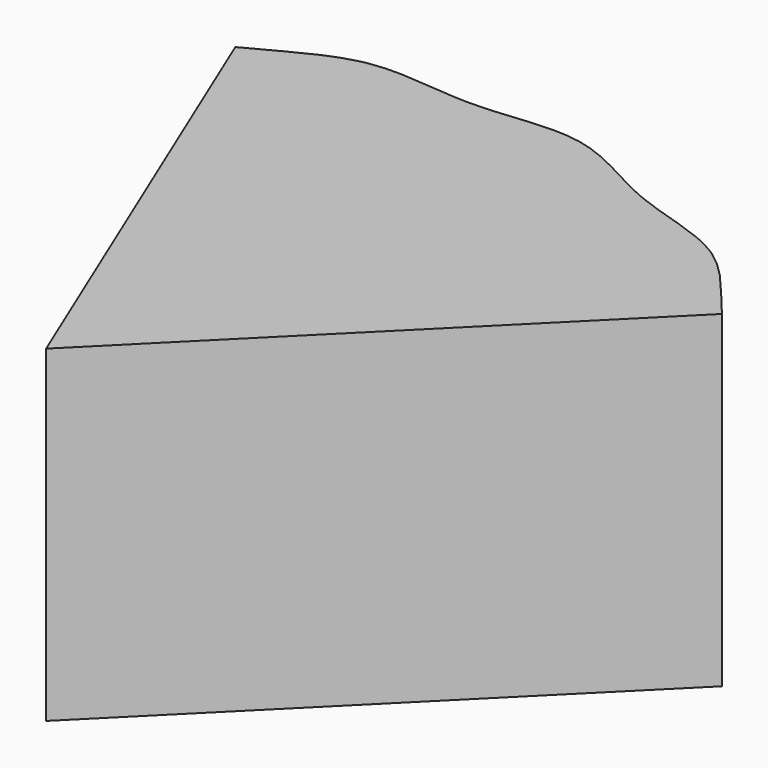
from build123d import *

# Parameters (mm, degrees)
F1_DEPTH = 25


# Not quite as in the source:
# - ends of sketch curves that miss each other by under 0.0002 mm in the source are joined


with BuildPart() as f1:
    # F0 (on Top) → F1 (new body)
    with BuildSketch(Plane.XY):
        with BuildLine():
            Line((-7.9011580417, 39.7218038563), (0, 0))
            Line((0, 0), (0, 40.5))
            ThreePointArc((0, 40.5), (-0.0234209669, 40.4999932279), (-0.046841926, 40.4999729115))
            ThreePointArc((-0.046841926, 40.4999729115), (-3.9930017081, 40.3026790345), (-7.9011580417, 39.7218038563))
        make_face()
        with BuildLine():
            Line((-15.4986790108, 37.4171210667), (0, 0))
            Line((0, 0), (-7.9011580417, 39.7218038563))
            ThreePointArc((-7.9011580417, 39.7218038563), (-11.7565294288, 38.7560835972), (-15.4986790108, 37.4171210667))
        make_face()
        with BuildLine():
            Line((22.5005944373, 33.6745192983), (0, 0))
            Line((0, 0), (28.6378246381, 28.6378246381))
            ThreePointArc((28.6378246381, 28.6378246381), (25.6929280086, 31.3069233612), (22.5005944373, 33.6745192983))
        make_face()
        with BuildLine():
            Line((15.4986790108, 37.4171210667), (0, 0))
            Line((0, 0), (22.5005944373, 33.6745192983))
            ThreePointArc((22.5005944373, 33.6745192983), (19.1122200978, 35.7067646663), (15.5419449411, 37.3991704112))
            ThreePointArc((15.5419449411, 37.3991704112), (15.5203145712, 37.4081519941), (15.4986790108, 37.4171210667))
        make_face()
        with BuildLine():
            Line((7.9011580417, 39.7218038563), (0, 0))
            Line((0, 0), (15.4986790108, 37.4171210667))
            ThreePointArc((15.4986790108, 37.4171210667), (11.7565294288, 38.7560835972), (7.9011580417, 39.7218038563))
        make_face()
        with BuildLine():
            Line((0, 40.5), (0, 0))
            Line((0, 0), (7.9011580417, 39.7218038563))
            ThreePointArc((7.9011580417, 39.7218038563), (3.9696941833, 40.3049814302), (0, 40.5))
        make_face()
        with BuildLine():
            add(Edge.make_bspline(
                [(0, 40.5), (2.7706806954, 40.5108669818), (5.5531529278, 41.2084422704), (8.0962483637, 40.7025891367)],
                knots=[0.375, 0.375, 0.375, 0.375, 0.5, 0.5, 0.5, 0.5], degree=3))
            ThreePointArc((0, 40.5), (3.9696941833, 40.3049814302), (7.9011580417, 39.7218038563))
            Line((7.9011580417, 39.7218038563), (8.0962483637, 40.7025891367))
        make_face()
        with BuildLine():
            ThreePointArc((-15.4986790108, 37.4171210667), (-11.7565294288, 38.7560835972), (-7.9011580417, 39.7218038563))
            Line((-7.9011580417, 39.7218038563), (-8.0962483637, 40.7025891367))
            ThreePointArc((-8.0962483637, 40.7025891367), (-8.3021528679, 40.6610902185), (-8.5078446962, 40.6185496864))
            add(Edge.make_bspline(
                [(-15.4986790108, 37.4171210667), (-13.169476805, 38.5739896459), (-10.9180232176, 40.0695028236), (-8.5078446962, 40.6185496864)],
                knots=[0.125, 0.125, 0.125, 0.125, 0.2432920147, 0.2432920147, 0.2432920147, 0.2432920147], degree=3))
        make_face()
        with BuildLine():
            Line((-8.0962483637, 40.7025891367), (-7.9011580417, 39.7218038563))
            ThreePointArc((-7.9011580417, 39.7218038563), (-3.9930017081, 40.3026790345), (-0.046841926, 40.4999729115))
            add(Edge.make_bspline(
                [(-8.0962483637, 40.7025891367), (-5.5440345136, 41.1623685455), (-2.801770338, 40.4967143515), (-0.046841926, 40.4999729115)],
                knots=[0.25, 0.25, 0.25, 0.25, 0.3742955555, 0.3742955555, 0.3742955555, 0.3742955555], degree=3))
        make_face()
        with BuildLine():
            ThreePointArc((22.5005944373, 33.6745192983), (25.6929280086, 31.3069233612), (28.6378246381, 28.6378246381))
            add(Edge.make_bspline(
                [(23.4042695923, 34.2708354852), (25.4208730599, 32.841246937), (26.9286368317, 30.597978935), (28.6378246381, 28.6378246381)],
                knots=[0.7567079853, 0.7567079853, 0.7567079853, 0.7567079853, 0.875, 0.875, 0.875, 0.875], degree=3))
            ThreePointArc((23.4042695923, 34.2708354852), (23.230514679, 34.388852667), (23.0561646703, 34.5059889106))
            Line((23.0561646703, 34.5059889106), (22.5005944373, 33.6745192983))
        make_face()
        with BuildLine():
            ThreePointArc((15.5419449411, 37.3991704112), (19.1122200978, 35.7067646663), (22.5005944373, 33.6745192983))
            Line((22.5005944373, 33.6745192983), (23.0561646703, 34.5059889106))
            add(Edge.make_bspline(
                [(15.5419449411, 37.3991704112), (18.0859199176, 36.3418944337), (20.8741764939, 35.907459652), (23.0561646703, 34.5059889106)],
                knots=[0.6257044445, 0.6257044445, 0.6257044445, 0.6257044445, 0.75, 0.75, 0.75, 0.75], degree=3))
        make_face()
        with BuildLine():
            ThreePointArc((7.9011580417, 39.7218038563), (11.7565294288, 38.7560835972), (15.4986790108, 37.4171210667))
            add(Edge.make_bspline(
                [(8.0962483637, 40.7025891367), (10.6393437996, 40.1967360031), (12.9430624391, 38.4874544473), (15.4986790108, 37.4171210667)],
                knots=[0.5, 0.5, 0.5, 0.5, 0.625, 0.625, 0.625, 0.625], degree=3))
            Line((8.0962483637, 40.7025891367), (7.9011580417, 39.7218038563))
        make_face()
    extrude(amount=F1_DEPTH)


solid = f1.part
